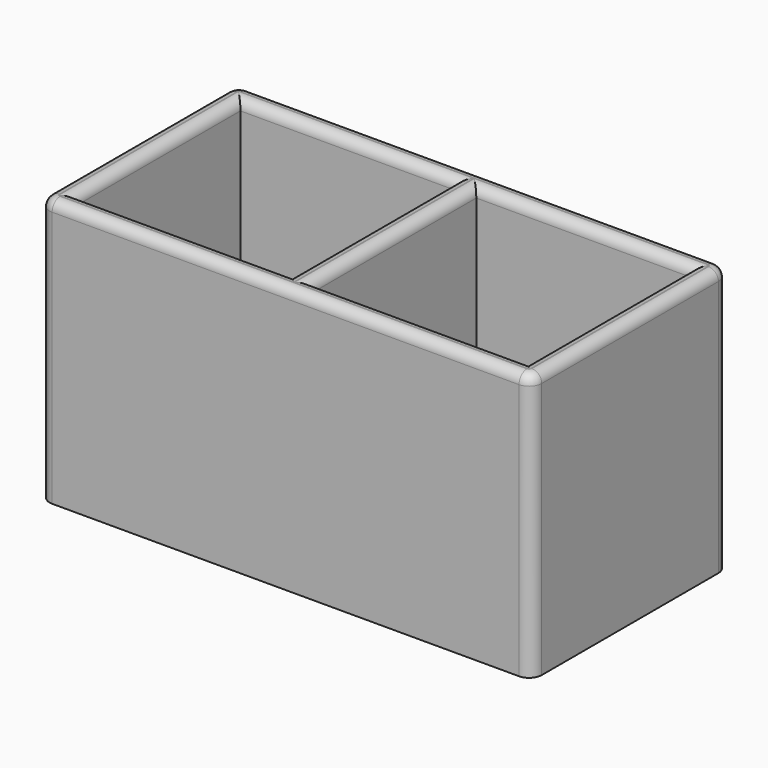
from build123d import *

# Parameters (mm, degrees)
F0_W         = 152.4
F0_H         = 76.2
F1_DEPTH     = 6.35
F2_W         = 152.4
F2_H         = 76.2
F2_W_2       = 66.675
F2_H_2       = 63.5
F3_DEPTH     = 76.2
F4_R         = 3.048
F5_T1_DEPTH  = 92.329
F5_T4_ANGLE  = 90
F5_T6_ANGLE  = 90
F5_T8_ANGLE  = 90
F5_T10_ANGLE = 90


# Not quite as in the source:
# - a fillet or chamfer that OpenCascade refuses, or shapes differently, is made with other operations: its cross-section is extruded or revolved along the edge and cut away or added
# - a feature names something its author has since deleted; it is built from what else it names


with BuildPart() as f1:
    # F0 (on Top) → F1 (new body)
    with BuildSketch(Plane.XY):
        with Locations((-119.875261867, -15.1447099686)):
            Rectangle(F0_W, F0_H)
    extrude(amount=F1_DEPTH)

    # F2 (on face) → F3 (join)
    with BuildSketch(Plane.XY.offset(6.35)):
        with Locations((-119.875261867, -15.1447099686)):
            Rectangle(F2_W, F2_H)
        with Locations((-156.387761867, -15.1447099686)):
            Rectangle(F2_W_2, F2_H_2, mode=Mode.SUBTRACT)
        with Locations((-83.362761867, -15.1447099686)):
            Rectangle(F2_W_2, F2_H_2, mode=Mode.SUBTRACT)
    extrude(amount=F3_DEPTH)

    # F4
    f4_edges = [f1.edges().sort_by_distance(p)[0] for p in [
        (-196.075262, -15.14471, 82.55),
        (-119.875262, 22.95529, 82.55),
        (-43.675262, -15.14471, 82.55),
        (-119.875262, -53.24471, 82.55),
        (-123.050262, -15.14471, 82.55),
        (-156.387762, -46.89471, 82.55),
        (-189.725262, -15.14471, 82.55),
        (-156.387762, 16.60529, 82.55),
        (-83.362762, 16.60529, 82.55),
        (-50.025262, -15.14471, 82.55),
        (-83.362762, -46.89471, 82.55),
        (-116.700262, -15.14471, 82.55),
    ]]
    fillet(f4_edges, radius=F4_R)

    # F5: fillet of radius 3.9116 on 4 edges, made by hand

    # F5_s2 → F5_t1 (cut)
    with BuildSketch(Plane.XY.offset(-9.779)):
        with BuildLine():
            ThreePointArc((-47.586861867, -53.2447099686), (-44.8209429818, -52.0990288539), (-43.675261867, -49.3331099686))
            Line((-43.675261867, -49.3331099686), (-43.675261867, -53.2447099686))
            Line((-43.675261867, -53.2447099686), (-47.586861867, -53.2447099686))
        make_face()
        with BuildLine():
            ThreePointArc((-43.675261867, 19.0436900314), (-44.8209429818, 21.8096089167), (-47.586861867, 22.9552900314))
            Line((-47.586861867, 22.9552900314), (-43.675261867, 22.9552900314))
            Line((-43.675261867, 22.9552900314), (-43.675261867, 19.0436900314))
        make_face()
        with BuildLine():
            ThreePointArc((-192.163661867, -53.2447099686), (-194.9295807523, -52.0990288539), (-196.075261867, -49.3331099686))
            Line((-196.075261867, -49.3331099686), (-196.075261867, -53.2447099686))
            Line((-196.075261867, -53.2447099686), (-192.163661867, -53.2447099686))
        make_face()
        with BuildLine():
            ThreePointArc((-196.075261867, 19.0436900314), (-194.9295807523, 21.8096089167), (-192.163661867, 22.9552900314))
            Line((-192.163661867, 22.9552900314), (-196.075261867, 22.9552900314))
            Line((-196.075261867, 22.9552900314), (-196.075261867, 19.0436900314))
        make_face()
    extrude(amount=F5_T1_DEPTH, mode=Mode.SUBTRACT)

    # F5_s3 → F5_t4 (revolve, cut)
    with BuildSketch(Plane.YZ.offset(-192.163661867)):
        with BuildLine():
            ThreePointArc((19.9072900314, 82.55), (22.0625515005, 81.6572614691), (22.9552900314, 79.502))
            Line((22.9552900314, 79.502), (22.9552900314, 82.55))
            Line((22.9552900314, 82.55), (19.9072900314, 82.55))
        make_face()
    revolve(axis=Axis((-192.163661867, 19.0436900314, 82.55), (0, 0, 1)), revolution_arc=F5_T4_ANGLE, mode=Mode.SUBTRACT)

    # F5_s5 → F5_t6 (revolve, cut)
    with BuildSketch(Plane.XZ.offset(49.3331099686)):
        with BuildLine():
            ThreePointArc((-193.027261867, 82.55), (-195.1825233361, 81.6572614691), (-196.075261867, 79.502))
            Line((-196.075261867, 79.502), (-196.075261867, 82.55))
            Line((-196.075261867, 82.55), (-193.027261867, 82.55))
        make_face()
    revolve(axis=Axis((-192.163661867, -49.3331099686, 82.55), (0, 0, 1)), revolution_arc=F5_T6_ANGLE, mode=Mode.SUBTRACT)

    # F5_s7 → F5_t8 (revolve, cut)
    with BuildSketch(Plane.XZ.offset(-19.0436900314)):
        with BuildLine():
            ThreePointArc((-46.723261867, 82.55), (-44.568000398, 81.6572614691), (-43.675261867, 79.502))
            Line((-43.675261867, 79.502), (-43.675261867, 82.55))
            Line((-43.675261867, 82.55), (-46.723261867, 82.55))
        make_face()
    revolve(axis=Axis((-47.586861867, 19.0436900314, 82.55), (0, 0, 1)), revolution_arc=F5_T8_ANGLE, mode=Mode.SUBTRACT)

    # F5_s9 → F5_t10 (revolve, cut)
    with BuildSketch(Plane.YZ.offset(-47.586861867)):
        with BuildLine():
            ThreePointArc((-50.1967099686, 82.55), (-52.3519714376, 81.6572614691), (-53.2447099686, 79.502))
            Line((-53.2447099686, 79.502), (-53.2447099686, 82.55))
            Line((-53.2447099686, 82.55), (-50.1967099686, 82.55))
        make_face()
    revolve(axis=Axis((-47.586861867, -49.3331099686, 82.55), (0, 0, 1)), revolution_arc=F5_T10_ANGLE, mode=Mode.SUBTRACT)


solid = f1.part
